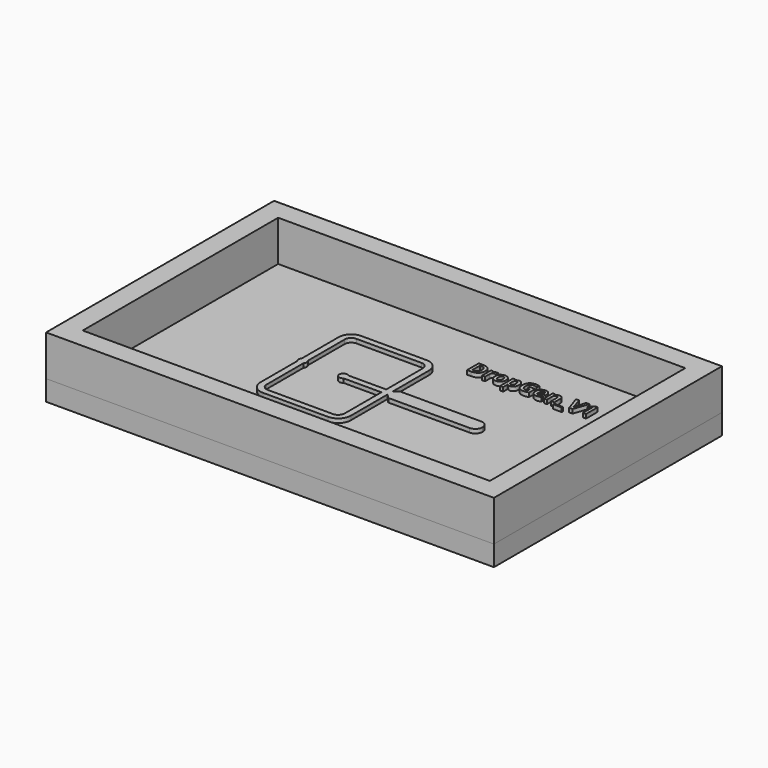
from build123d import *

# Parameters (mm, degrees)
F0_W         = 55
F0_H         = 35
F0_W_2       = 50
F0_H_2       = 30
F1_DEPTH     = 5
F2_DEPTH     = 2.5
F3_DEPTH     = 0.5
F0_TEXT_SIZE = 2.5179007003
F4_DEPTH     = 0.5
F0_W_3       = 1.0453222126
F0_H_3       = 0.1723188292
F5_DEPTH     = 2.5


# Not quite as in the source:
# - Text() gives the source's letters only with a copy of the font that has no kerning and outlines rounded to 1/6400 em; it was checked with that copy


with BuildPart() as f1:
    # F0 (on Top) → F1 (new body)
    with BuildSketch(Plane.XY):
        Rectangle(F0_W, F0_H)
        Rectangle(F0_W_2, F0_H_2, mode=Mode.SUBTRACT)
    extrude(amount=F1_DEPTH)

    # F0 (on Top) → F2 (join)
    with BuildSketch(Plane.XY):
        Rectangle(F0_W, F0_H)
        Rectangle(F0_W_2, F0_H_2, mode=Mode.SUBTRACT)
    extrude(amount=-F2_DEPTH)


with BuildPart() as f3:
    # F0 (on Top) → F3 (new body)
    with BuildSketch(Plane.XY):
        with BuildLine():
            ThreePointArc((-8.825, 7.55), (-9.9210155108, 7.0960155108), (-10.375, 6))
            Line((-10.375, 6), (-10.375, 0.3307189139))
            ThreePointArc((-10.375, 0.3307189139), (-10.5, 0), (-10.375, -0.3307189139))
            Line((-10.375, -0.3307189139), (-10.375, -6))
            ThreePointArc((-10.375, -6), (-9.9210155108, -7.0960155108), (-8.825, -7.55))
            Line((-8.825, -7.55), (-0.825, -7.55))
            ThreePointArc((-0.825, -7.55), (0.2710155108, -7.0960155108), (0.725, -6))
            Line((0.725, -6), (0.725, -0.375))
            Line((0.725, -0.375), (1.225, -0.875))
            Line((1.225, -0.875), (11.225, -0.875))
            ThreePointArc((11.225, -0.875), (10.35, 0), (11.225, 0.875))
            Line((11.225, 0.875), (1.225, 0.875))
            Line((1.225, 0.875), (0.725, 0.375))
            Line((0.725, 0.375), (0.725, 6))
            ThreePointArc((0.725, 6), (0.2710155108, 7.0960155108), (-0.825, 7.55))
            Line((-0.825, 7.55), (-8.825, 7.55))
        make_face()
        with BuildLine():
            Line((-9.625, 0.3307189139), (-9.625, 6))
            ThreePointArc((-9.625, 6), (-9.3906854249, 6.5656854249), (-8.825, 6.8))
            Line((-8.825, 6.8), (-0.825, 6.8))
            ThreePointArc((-0.825, 6.8), (-0.2593145751, 6.5656854249), (-0.025, 6))
            Line((-0.025, 6), (-0.025, 0.375))
            Line((-0.025, 0.375), (-4.6692810861, 0.375))
            ThreePointArc((-4.6692810861, 0.375), (-5.5, 0), (-4.6692810861, -0.375))
            Line((-4.6692810861, -0.375), (-0.025, -0.375))
            Line((-0.025, -0.375), (-0.025, -6))
            ThreePointArc((-0.025, -6), (-0.2593145751, -6.5656854249), (-0.825, -6.8))
            Line((-0.825, -6.8), (-8.825, -6.8))
            ThreePointArc((-8.825, -6.8), (-9.3906854249, -6.5656854249), (-9.625, -6))
            Line((-9.625, -6), (-9.625, -0.3307189139))
            ThreePointArc((-9.625, -0.3307189139), (-9.5, 0), (-9.625, 0.3307189139))
        make_face(mode=Mode.SUBTRACT)
        with BuildLine():
            ThreePointArc((12.1, 0), (11.8437184335, 0.6187184335), (11.225, 0.875))
            ThreePointArc((11.225, 0.875), (10.35, 0), (11.225, -0.875))
            ThreePointArc((11.225, -0.875), (11.8437184335, -0.6187184335), (12.1, 0))
        make_face()
    extrude(amount=F3_DEPTH)


with BuildPart() as f4:
    # F0 (on Top) → F4 (new body)
    with BuildSketch(Plane.XY):
        with Locations((3.2864760142, 8.3606809292)):
            Text('DropGen_V1', F0_TEXT_SIZE, font='Open Sans', font_style=FontStyle.BOLD, text_align=(TextAlign.LEFT, TextAlign.BOTTOM))
    extrude(amount=F4_DEPTH)


with BuildPart() as f5:
    # F0 (on Top) → F5 (new body)
    with BuildSketch(Plane.XY):
        Rectangle(F0_W, F0_H)
        Rectangle(F0_W_2, F0_H_2, mode=Mode.SUBTRACT)
        Rectangle(F0_W_2, F0_H_2)
        with BuildLine():
            Line((-10.375, 0.3307189139), (-10.375, 6))
            ThreePointArc((-10.375, 6), (-9.9210155108, 7.0960155108), (-8.825, 7.55))
            Line((-8.825, 7.55), (-0.825, 7.55))
            ThreePointArc((-0.825, 7.55), (0.2710155108, 7.0960155108), (0.725, 6))
            Line((0.725, 6), (0.725, 0.375))
            Line((0.725, 0.375), (1.225, 0.875))
            Line((1.225, 0.875), (11.225, 0.875))
            ThreePointArc((11.225, 0.875), (11.8437184335, 0.6187184335), (12.1, 0))
            ThreePointArc((12.1, 0), (11.8437184335, -0.6187184335), (11.225, -0.875))
            Line((11.225, -0.875), (1.225, -0.875))
            Line((1.225, -0.875), (0.725, -0.375))
            Line((0.725, -0.375), (0.725, -6))
            ThreePointArc((0.725, -6), (0.2710155108, -7.0960155108), (-0.825, -7.55))
            Line((-0.825, -7.55), (-8.825, -7.55))
            ThreePointArc((-8.825, -7.55), (-9.9210155108, -7.0960155108), (-10.375, -6))
            Line((-10.375, -6), (-10.375, -0.3307189139))
            ThreePointArc((-10.375, -0.3307189139), (-10.5, 0), (-10.375, 0.3307189139))
        make_face(mode=Mode.SUBTRACT)
        with Locations((14.9292095101, 8.0483038736)):
            Rectangle(F0_W_3, F0_H_3, mode=Mode.SUBTRACT)
        with BuildLine():
            add(Edge.make_bspline(
                [(4.7606281898, 9.9259102942), (5.0041563982, 9.6935946124), (5.0041563982, 9.2765673089)],
                knots=[0, 0, 0, 1, 1, 1], degree=2))
            add(Edge.make_bspline(
                [(5.0041563982, 9.2765673089), (5.0041563982, 8.8327873105), (4.7513827732, 8.5967341198)],
                knots=[0, 0, 0, 1, 1, 1], degree=2))
            add(Edge.make_bspline(
                [(4.7513827732, 8.5967341198), (4.4986091482, 8.3606809292), (4.0217817031, 8.3606809292)],
                knots=[0, 0, 0, 1, 1, 1], degree=2))
            Line((4.0217817031, 8.3606809292), (3.5126936552, 8.3606809292))
            Line((3.5126936552, 8.3606809292), (3.5126936552, 10.158225976))
            Line((3.5126936552, 10.158225976), (4.0768607809, 10.158225976))
            add(Edge.make_bspline(
                [(4.0768607809, 10.158225976), (4.5170999814, 10.158225976), (4.7606281898, 9.9259102942)],
                knots=[0, 0, 0, 1, 1, 1], degree=2))
        make_face(mode=Mode.SUBTRACT)
        with BuildLine():
            add(Edge.make_bspline(
                [(5.8777499146, 9.6902505255), (5.9865310933, 9.7608697717), (6.1143932382, 9.7608697717)],
                knots=[0, 0, 0, 1, 1, 1], degree=2))
            add(Edge.make_bspline(
                [(6.1143932382, 9.7608697717), (6.1907171032, 9.7608697717), (6.2410751172, 9.7498539562)],
                knots=[0, 0, 0, 1, 1, 1], degree=2))
            Line((6.2410751172, 9.7498539562), (6.2127487343, 9.3985281241))
            add(Edge.make_bspline(
                [(6.2127487343, 9.3985281241), (6.1671117841, 9.4107242056), (6.1021971567, 9.4107242056)],
                knots=[0, 0, 0, 1, 1, 1], degree=2))
            add(Edge.make_bspline(
                [(6.1021971567, 9.4107242056), (5.9227967318, 9.4107242056), (5.8224741258, 9.3184667503)],
                knots=[0, 0, 0, 1, 1, 1], degree=2))
            add(Edge.make_bspline(
                [(5.8224741258, 9.3184667503), (5.7221515197, 9.2262092949), (5.7221515197, 9.0601852175)],
                knots=[0, 0, 0, 1, 1, 1], degree=2))
            Line((5.7221515197, 9.0601852175), (5.7221515197, 8.3606809292))
            Line((5.7221515197, 8.3606809292), (5.3472203686, 8.3606809292))
            Line((5.3472203686, 8.3606809292), (5.3472203686, 9.7352973427))
            Line((5.3472203686, 9.7352973427), (5.6312710413, 9.7352973427))
            Line((5.6312710413, 9.7352973427), (5.6867435411, 9.5039652159))
            Line((5.6867435411, 9.5039652159), (5.7048409524, 9.5039652159))
            add(Edge.make_bspline(
                [(5.7048409524, 9.5039652159), (5.7689687359, 9.6196312793), (5.8777499146, 9.6902505255)],
                knots=[0, 0, 0, 1, 1, 1], degree=2))
        make_face(mode=Mode.SUBTRACT)
        with BuildLine():
            add(Edge.make_bspline(
                [(7.658574527, 9.4278380619), (7.7396194558, 9.2667317593), (7.7396194558, 9.0503496679)],
                knots=[0, 0, 0, 1, 1, 1], degree=2))
            add(Edge.make_bspline(
                [(7.7396194558, 9.0503496679), (7.7396194558, 8.7147607152), (7.5625795628, 8.5253280297)],
                knots=[0, 0, 0, 1, 1, 1], degree=2))
            add(Edge.make_bspline(
                [(7.5625795628, 8.5253280297), (7.3855396699, 8.3358953442), (7.0696218164, 8.3358953442)],
                knots=[0, 0, 0, 1, 1, 1], degree=2))
            add(Edge.make_bspline(
                [(7.0696218164, 8.3358953442), (6.8717305582, 8.3358953442), (6.7204598052, 8.4226448917)],
                knots=[0, 0, 0, 1, 1, 1], degree=2))
            add(Edge.make_bspline(
                [(6.7204598052, 8.4226448917), (6.5691890522, 8.5093944393), (6.4881441234, 8.6716810079)],
                knots=[0, 0, 0, 1, 1, 1], degree=2))
            add(Edge.make_bspline(
                [(6.4881441234, 8.6716810079), (6.4070991946, 8.8339675764), (6.4070991946, 9.0503496679)],
                knots=[0, 0, 0, 1, 1, 1], degree=2))
            add(Edge.make_bspline(
                [(6.4070991946, 9.0503496679), (6.4070991946, 9.3871188865), (6.5827621106, 9.5739943291)],
                knots=[0, 0, 0, 1, 1, 1], degree=2))
            add(Edge.make_bspline(
                [(6.5827621106, 9.5739943291), (6.7584250267, 9.7608697717), (7.0770968341, 9.7608697717)],
                knots=[0, 0, 0, 1, 1, 1], degree=2))
            add(Edge.make_bspline(
                [(7.0770968341, 9.7608697717), (7.2749880922, 9.7608697717), (7.4262588452, 9.6749070681)],
                knots=[0, 0, 0, 1, 1, 1], degree=2))
            add(Edge.make_bspline(
                [(7.4262588452, 9.6749070681), (7.5775295983, 9.5889443645), (7.658574527, 9.4278380619)],
                knots=[0, 0, 0, 1, 1, 1], degree=2))
        make_face(mode=Mode.SUBTRACT)
        with BuildLine():
            add(Edge.make_bspline(
                [(9.0847292206, 8.4208744928), (8.9655223593, 8.3358953442), (8.8046127677, 8.3358953442)],
                knots=[0, 0, 0, 1, 1, 1], degree=2))
            add(Edge.make_bspline(
                [(8.8046127677, 8.3358953442), (8.5622648253, 8.3358953442), (8.4245671307, 8.5117549712)],
                knots=[0, 0, 0, 1, 1, 1], degree=2))
            Line((8.4245671307, 8.5117549712), (8.4048960315, 8.5117549712))
            add(Edge.make_bspline(
                [(8.4048960315, 8.5117549712), (8.4245671307, 8.339829564), (8.4245671307, 8.3126834471)],
                knots=[0, 0, 0, 1, 1, 1], degree=2))
            Line((8.4245671307, 8.3126834471), (8.4245671307, 7.7555979171))
            Line((8.4245671307, 7.7555979171), (8.0496359796, 7.7555979171))
            Line((8.0496359796, 7.7555979171), (8.0496359796, 9.7352973427))
            Line((8.0496359796, 9.7352973427), (8.3545380175, 9.7352973427))
            Line((8.3545380175, 9.7352973427), (8.4072565634, 9.5570771838))
            Line((8.4072565634, 9.5570771838), (8.4245671307, 9.5570771838))
            add(Edge.make_bspline(
                [(8.4245671307, 9.5570771838), (8.5563634955, 9.7608697717), (8.8144483173, 9.7608697717)],
                knots=[0, 0, 0, 1, 1, 1], degree=2))
            add(Edge.make_bspline(
                [(8.8144483173, 9.7608697717), (9.0579765256, 9.7608697717), (9.1956742202, 9.5728140632)],
                knots=[0, 0, 0, 1, 1, 1], degree=2))
            add(Edge.make_bspline(
                [(9.1956742202, 9.5728140632), (9.3333719147, 9.3847583546), (9.3333719147, 9.0503496679)],
                knots=[0, 0, 0, 1, 1, 1], degree=2))
            add(Edge.make_bspline(
                [(9.3333719147, 9.0503496679), (9.3333719147, 8.8304267786), (9.2686539983, 8.66814021)],
                knots=[0, 0, 0, 1, 1, 1], degree=2))
            add(Edge.make_bspline(
                [(9.2686539983, 8.66814021), (9.2039360819, 8.5058536414), (9.0847292206, 8.4208744928)],
                knots=[0, 0, 0, 1, 1, 1], degree=2))
        make_face(mode=Mode.SUBTRACT)
        with BuildLine():
            Line((10.3546953863, 9.0527101998), (10.3546953863, 9.3702017412))
            Line((10.3546953863, 9.3702017412), (11.067969444, 9.3702017412))
            Line((11.067969444, 9.3702017412), (11.067969444, 8.4381850601))
            add(Edge.make_bspline(
                [(11.067969444, 8.4381850601), (10.8944703489, 8.3815322944), (10.741429197, 8.3587138193)],
                knots=[0, 0, 0, 1, 1, 1], degree=2))
            add(Edge.make_bspline(
                [(10.741429197, 8.3587138193), (10.588388045, 8.3358953442), (10.4286587194, 8.3358953442)],
                knots=[0, 0, 0, 1, 1, 1], degree=2))
            add(Edge.make_bspline(
                [(10.4286587194, 8.3358953442), (10.0218603875, 8.3358953442), (9.807248695, 8.5750959107)],
                knots=[0, 0, 0, 1, 1, 1], degree=2))
            add(Edge.make_bspline(
                [(9.807248695, 8.5750959107), (9.5926370025, 8.8142964772), (9.5926370025, 9.2620106955)],
                knots=[0, 0, 0, 1, 1, 1], degree=2))
            add(Edge.make_bspline(
                [(9.5926370025, 9.2620106955), (9.5926370025, 9.6971354103), (9.8416731186, 9.9404669076)],
                knots=[0, 0, 0, 1, 1, 1], degree=2))
            add(Edge.make_bspline(
                [(9.8416731186, 9.9404669076), (10.0907092347, 10.183798405), (10.5317352793, 10.183798405)],
                knots=[0, 0, 0, 1, 1, 1], degree=2))
            add(Edge.make_bspline(
                [(10.5317352793, 10.183798405), (10.8087043563, 10.183798405), (11.0656089121, 10.0732468274)],
                knots=[0, 0, 0, 1, 1, 1], degree=2))
            Line((11.0656089121, 10.0732468274), (10.9389270331, 9.7683447894))
            add(Edge.make_bspline(
                [(10.9389270331, 9.7683447894), (10.7422160409, 9.8667002855), (10.5293747474, 9.8667002855)],
                knots=[0, 0, 0, 1, 1, 1], degree=2))
            add(Edge.make_bspline(
                [(10.5293747474, 9.8667002855), (10.2823057411, 9.8667002855), (10.133592231, 9.7006762081)],
                knots=[0, 0, 0, 1, 1, 1], degree=2))
            add(Edge.make_bspline(
                [(10.133592231, 9.7006762081), (9.9848787209, 9.5346521307), (9.9848787209, 9.2545356778)],
                knots=[0, 0, 0, 1, 1, 1], degree=2))
            add(Edge.make_bspline(
                [(9.9848787209, 9.2545356778), (9.9848787209, 8.9618297214), (10.1046757152, 8.8076083035)],
                knots=[0, 0, 0, 1, 1, 1], degree=2))
            add(Edge.make_bspline(
                [(10.1046757152, 8.8076083035), (10.2244727094, 8.6533868856), (10.4530508824, 8.6533868856)],
                knots=[0, 0, 0, 1, 1, 1], degree=2))
            add(Edge.make_bspline(
                [(10.4530508824, 8.6533868856), (10.5726511656, 8.6533868856), (10.6953988248, 8.6777790486)],
                knots=[0, 0, 0, 1, 1, 1], degree=2))
            Line((10.6953988248, 8.6777790486), (10.6953988248, 9.0527101998))
            Line((10.6953988248, 9.0527101998), (10.3546953863, 9.0527101998))
        make_face(mode=Mode.SUBTRACT)
        with BuildLine():
            add(Edge.make_bspline(
                [(12.3611475068, 8.3598940852), (12.2494156632, 8.3358953442), (12.0881126496, 8.3358953442)],
                knots=[0, 0, 0, 1, 1, 1], degree=2))
            add(Edge.make_bspline(
                [(12.0881126496, 8.3358953442), (11.7564579168, 8.3358953442), (11.5695824742, 8.5192299889)],
                knots=[0, 0, 0, 1, 1, 1], degree=2))
            add(Edge.make_bspline(
                [(11.5695824742, 8.5192299889), (11.3827070316, 8.7025646336), (11.3827070316, 9.0381535864)],
                knots=[0, 0, 0, 1, 1, 1], degree=2))
            add(Edge.make_bspline(
                [(11.3827070316, 9.0381535864), (11.3827070316, 9.3835780887), (11.5554192827, 9.5722239302)],
                knots=[0, 0, 0, 1, 1, 1], degree=2))
            add(Edge.make_bspline(
                [(11.5554192827, 9.5722239302), (11.7281315339, 9.7608697717), (12.0330335718, 9.7608697717)],
                knots=[0, 0, 0, 1, 1, 1], degree=2))
            add(Edge.make_bspline(
                [(12.0330335718, 9.7608697717), (12.3241658403, 9.7608697717), (12.4864524089, 9.5950424053)],
                knots=[0, 0, 0, 1, 1, 1], degree=2))
            add(Edge.make_bspline(
                [(12.4864524089, 9.5950424053), (12.6487389774, 9.4292150389), (12.6487389774, 9.1365090825)],
                knots=[0, 0, 0, 1, 1, 1], degree=2))
            Line((12.6487389774, 9.1365090825), (12.6487389774, 8.9543547037))
            Line((12.6487389774, 8.9543547037), (11.7623592465, 8.9543547037))
            add(Edge.make_bspline(
                [(11.7623592465, 8.9543547037), (11.7686539983, 8.794625378), (11.8571739448, 8.7049251655)],
                knots=[0, 0, 0, 1, 1, 1], degree=2))
            add(Edge.make_bspline(
                [(11.8571739448, 8.7049251655), (11.9456938913, 8.6152249531), (12.105423217, 8.6152249531)],
                knots=[0, 0, 0, 1, 1, 1], degree=2))
            add(Edge.make_bspline(
                [(12.105423217, 8.6152249531), (12.229744564, 8.6152249531), (12.3402961417, 8.6409940931)],
                knots=[0, 0, 0, 1, 1, 1], degree=2))
            add(Edge.make_bspline(
                [(12.3402961417, 8.6409940931), (12.4508477193, 8.6667632331), (12.5712348465, 8.7234159988)],
                knots=[0, 0, 0, 1, 1, 1], degree=2))
            Line((12.5712348465, 8.7234159988), (12.5712348465, 8.4330705743))
            add(Edge.make_bspline(
                [(12.5712348465, 8.4330705743), (12.4728793504, 8.3838928263), (12.3611475068, 8.3598940852)],
                knots=[0, 0, 0, 1, 1, 1], degree=2))
        make_face(mode=Mode.SUBTRACT)
        with BuildLine():
            Line((14.2224269151, 9.2568962097), (14.2224269151, 8.3606809292))
            Line((14.2224269151, 8.3606809292), (13.847495764, 8.3606809292))
            Line((13.847495764, 8.3606809292), (13.847495764, 9.1636551994))
            add(Edge.make_bspline(
                [(13.847495764, 9.1636551994), (13.847495764, 9.3123687095), (13.7945805071, 9.3867254646)],
                knots=[0, 0, 0, 1, 1, 1], degree=2))
            add(Edge.make_bspline(
                [(13.7945805071, 9.3867254646), (13.7416652502, 9.4610822196), (13.6259991867, 9.4610822196)],
                knots=[0, 0, 0, 1, 1, 1], degree=2))
            add(Edge.make_bspline(
                [(13.6259991867, 9.4610822196), (13.468630393, 9.4610822196), (13.3986012797, 9.3560385498)],
                knots=[0, 0, 0, 1, 1, 1], degree=2))
            add(Edge.make_bspline(
                [(13.3986012797, 9.3560385498), (13.3285721665, 9.2509948799), (13.3285721665, 9.0074666716)],
                knots=[0, 0, 0, 1, 1, 1], degree=2))
            Line((13.3285721665, 9.0074666716), (13.3285721665, 8.3606809292))
            Line((13.3285721665, 8.3606809292), (12.9536410154, 8.3606809292))
            Line((12.9536410154, 8.3606809292), (12.9536410154, 9.7352973427))
            Line((12.9536410154, 9.7352973427), (13.24005222, 9.7352973427))
            Line((13.24005222, 9.7352973427), (13.290410234, 9.5594377157))
            Line((13.290410234, 9.5594377157), (13.3112615992, 9.5594377157))
            add(Edge.make_bspline(
                [(13.3112615992, 9.5594377157), (13.3742091167, 9.6589734778), (13.4841705614, 9.7099216248)],
                knots=[0, 0, 0, 1, 1, 1], degree=2))
            add(Edge.make_bspline(
                [(13.4841705614, 9.7099216248), (13.594132006, 9.7608697717), (13.7341902325, 9.7608697717)],
                knots=[0, 0, 0, 1, 1, 1], degree=2))
            add(Edge.make_bspline(
                [(13.7341902325, 9.7608697717), (13.9741776429, 9.7608697717), (14.098302279, 9.6312372279)],
                knots=[0, 0, 0, 1, 1, 1], degree=2))
            add(Edge.make_bspline(
                [(14.098302279, 9.6312372279), (14.2224269151, 9.501604684), (14.2224269151, 9.2568962097)],
                knots=[0, 0, 0, 1, 1, 1], degree=2))
        make_face(mode=Mode.SUBTRACT)
        with BuildLine():
            Line((16.3579214466, 9.0885116004), (16.6982314631, 10.158225976))
            Line((16.6982314631, 10.158225976), (17.0829981638, 10.158225976))
            Line((17.0829981638, 10.158225976), (16.472013822, 8.3606809292))
            Line((16.472013822, 8.3606809292), (16.0565602065, 8.3606809292))
            Line((16.0565602065, 8.3606809292), (15.4467561306, 10.158225976))
            Line((15.4467561306, 10.158225976), (15.8315228314, 10.158225976))
            Line((15.8315228314, 10.158225976), (16.169865738, 9.0885116004))
            add(Edge.make_bspline(
                [(16.169865738, 9.0885116004), (16.1977986989, 8.9936969021), (16.2280921917, 8.8678018671)],
                knots=[0, 0, 0, 1, 1, 1], degree=2))
            add(Edge.make_bspline(
                [(16.2280921917, 8.8678018671), (16.2583856845, 8.7419068321), (16.2654672802, 8.692729084)],
                knots=[0, 0, 0, 1, 1, 1], degree=2))
            add(Edge.make_bspline(
                [(16.2654672802, 8.692729084), (16.2792370497, 8.8056411936), (16.3579214466, 9.0885116004)],
                knots=[0, 0, 0, 1, 1, 1], degree=2))
        make_face(mode=Mode.SUBTRACT)
        with BuildLine():
            Line((18.1232058906, 10.158225976), (18.1232058906, 8.3606809292))
            Line((18.1232058906, 8.3606809292), (17.7431602537, 8.3606809292))
            Line((17.7431602537, 8.3606809292), (17.7431602537, 9.400888656))
            Line((17.7431602537, 9.400888656), (17.7470944735, 9.5716337972))
            Line((17.7470944735, 9.5716337972), (17.7529958033, 9.7585092398))
            add(Edge.make_bspline(
                [(17.7529958033, 9.7585092398), (17.658574527, 9.6640879636), (17.6215928605, 9.6345813147)],
                knots=[0, 0, 0, 1, 1, 1], degree=2))
            Line((17.6215928605, 9.6345813147), (17.4150463187, 9.4685572373))
            Line((17.4150463187, 9.4685572373), (17.231711674, 9.6971354103))
            Line((17.231711674, 9.6971354103), (17.810828835, 10.158225976))
            Line((17.810828835, 10.158225976), (18.1232058906, 10.158225976))
        make_face(mode=Mode.SUBTRACT)
        with BuildLine():
            ThreePointArc((-8.825, 7.55), (-9.9210155108, 7.0960155108), (-10.375, 6))
            Line((-10.375, 6), (-10.375, 0.3307189139))
            ThreePointArc((-10.375, 0.3307189139), (-10.5, 0), (-10.375, -0.3307189139))
            Line((-10.375, -0.3307189139), (-10.375, -6))
            ThreePointArc((-10.375, -6), (-9.9210155108, -7.0960155108), (-8.825, -7.55))
            Line((-8.825, -7.55), (-0.825, -7.55))
            ThreePointArc((-0.825, -7.55), (0.2710155108, -7.0960155108), (0.725, -6))
            Line((0.725, -6), (0.725, -0.375))
            Line((0.725, -0.375), (1.225, -0.875))
            Line((1.225, -0.875), (11.225, -0.875))
            ThreePointArc((11.225, -0.875), (10.35, 0), (11.225, 0.875))
            Line((11.225, 0.875), (1.225, 0.875))
            Line((1.225, 0.875), (0.725, 0.375))
            Line((0.725, 0.375), (0.725, 6))
            ThreePointArc((0.725, 6), (0.2710155108, 7.0960155108), (-0.825, 7.55))
            Line((-0.825, 7.55), (-8.825, 7.55))
        make_face()
        with BuildLine():
            Line((-9.625, 0.3307189139), (-9.625, 6))
            ThreePointArc((-9.625, 6), (-9.3906854249, 6.5656854249), (-8.825, 6.8))
            Line((-8.825, 6.8), (-0.825, 6.8))
            ThreePointArc((-0.825, 6.8), (-0.2593145751, 6.5656854249), (-0.025, 6))
            Line((-0.025, 6), (-0.025, 0.375))
            Line((-0.025, 0.375), (-4.6692810861, 0.375))
            ThreePointArc((-4.6692810861, 0.375), (-5.5, 0), (-4.6692810861, -0.375))
            Line((-4.6692810861, -0.375), (-0.025, -0.375))
            Line((-0.025, -0.375), (-0.025, -6))
            ThreePointArc((-0.025, -6), (-0.2593145751, -6.5656854249), (-0.825, -6.8))
            Line((-0.825, -6.8), (-8.825, -6.8))
            ThreePointArc((-8.825, -6.8), (-9.3906854249, -6.5656854249), (-9.625, -6))
            Line((-9.625, -6), (-9.625, -0.3307189139))
            ThreePointArc((-9.625, -0.3307189139), (-9.5, 0), (-9.625, 0.3307189139))
        make_face(mode=Mode.SUBTRACT)
        with BuildLine():
            ThreePointArc((-8.825, 6.8), (-9.3906854249, 6.5656854249), (-9.625, 6))
            Line((-9.625, 6), (-9.625, 0.3307189139))
            ThreePointArc((-9.625, 0.3307189139), (-9.5, 0), (-9.625, -0.3307189139))
            Line((-9.625, -0.3307189139), (-9.625, -6))
            ThreePointArc((-9.625, -6), (-9.3906854249, -6.5656854249), (-8.825, -6.8))
            Line((-8.825, -6.8), (-0.825, -6.8))
            ThreePointArc((-0.825, -6.8), (-0.2593145751, -6.5656854249), (-0.025, -6))
            Line((-0.025, -6), (-0.025, -0.375))
            Line((-0.025, -0.375), (-4.6692810861, -0.375))
            ThreePointArc((-4.6692810861, -0.375), (-5.5, 0), (-4.6692810861, 0.375))
            Line((-4.6692810861, 0.375), (-0.025, 0.375))
            Line((-0.025, 0.375), (-0.025, 6))
            ThreePointArc((-0.025, 6), (-0.2593145751, 6.5656854249), (-0.825, 6.8))
            Line((-0.825, 6.8), (-8.825, 6.8))
        make_face()
        with BuildLine():
            ThreePointArc((12.1, 0), (11.8437184335, 0.6187184335), (11.225, 0.875))
            ThreePointArc((11.225, 0.875), (10.35, 0), (11.225, -0.875))
            ThreePointArc((11.225, -0.875), (11.8437184335, -0.6187184335), (12.1, 0))
        make_face()
        with BuildLine():
            add(Edge.make_bspline(
                [(5.0041563982, 9.2765673089), (5.0041563982, 8.8327873105), (4.7513827732, 8.5967341198)],
                knots=[0, 0, 0, 1, 1, 1], degree=2))
            add(Edge.make_bspline(
                [(4.7606281898, 9.9259102942), (5.0041563982, 9.6935946124), (5.0041563982, 9.2765673089)],
                knots=[0, 0, 0, 1, 1, 1], degree=2))
            add(Edge.make_bspline(
                [(4.0768607809, 10.158225976), (4.5170999814, 10.158225976), (4.7606281898, 9.9259102942)],
                knots=[0, 0, 0, 1, 1, 1], degree=2))
            Line((4.0768607809, 10.158225976), (3.5126936552, 10.158225976))
            Line((3.5126936552, 10.158225976), (3.5126936552, 8.3606809292))
            Line((3.5126936552, 8.3606809292), (4.0217817031, 8.3606809292))
            add(Edge.make_bspline(
                [(4.7513827732, 8.5967341198), (4.4986091482, 8.3606809292), (4.0217817031, 8.3606809292)],
                knots=[0, 0, 0, 1, 1, 1], degree=2))
        make_face()
        with BuildLine():
            add(Edge.make_bspline(
                [(4.6079804599, 9.2667317593), (4.6079804599, 9.8458489204), (4.0965318801, 9.8458489204)],
                knots=[0, 0, 0, 1, 1, 1], degree=2))
            add(Edge.make_bspline(
                [(4.0571896817, 8.6754185167), (4.6079804599, 8.6754185167), (4.6079804599, 9.2667317593)],
                knots=[0, 0, 0, 1, 1, 1], degree=2))
            Line((4.0571896817, 8.6754185167), (3.8939195581, 8.6754185167))
            Line((3.8939195581, 8.6754185167), (3.8939195581, 9.8458489204))
            Line((3.8939195581, 9.8458489204), (4.0965318801, 9.8458489204))
        make_face(mode=Mode.SUBTRACT)
        with BuildLine():
            add(Edge.make_bspline(
                [(4.0571896817, 8.6754185167), (4.6079804599, 8.6754185167), (4.6079804599, 9.2667317593)],
                knots=[0, 0, 0, 1, 1, 1], degree=2))
            add(Edge.make_bspline(
                [(4.6079804599, 9.2667317593), (4.6079804599, 9.8458489204), (4.0965318801, 9.8458489204)],
                knots=[0, 0, 0, 1, 1, 1], degree=2))
            Line((4.0965318801, 9.8458489204), (3.8939195581, 9.8458489204))
            Line((3.8939195581, 9.8458489204), (3.8939195581, 8.6754185167))
            Line((3.8939195581, 8.6754185167), (4.0571896817, 8.6754185167))
        make_face()
    extrude(amount=-F5_DEPTH)


solid = Compound([f1.part, f3.part, f4.part, f5.part])
